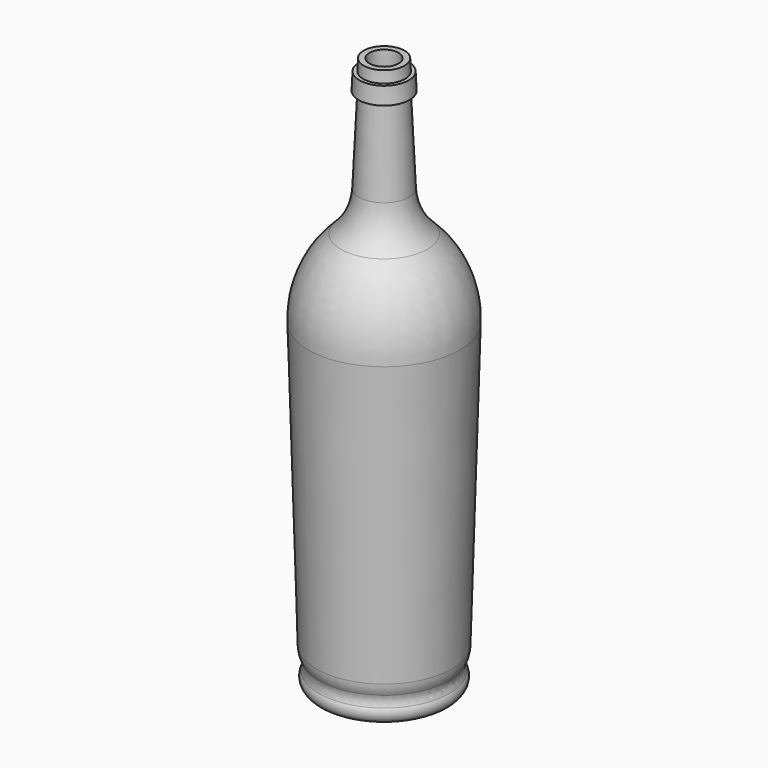
from build123d import *

# Parameters (mm, degrees)
F2_R = 1
F3_T = -0.5


with BuildPart() as f1:
    # F0 (on Front) → F1 (revolve)
    with BuildSketch(Plane.XZ):
        with BuildLine():
            Line((1.744893219, 47.2681485116), (0, 47.2681485116))
            Line((0, 47.2681485116), (0, 0))
            Line((0, 0), (5.1215616986, 0))
            ThreePointArc((5.1215616986, 0), (5.6702853456, 0.8186125558), (5.1215616986, 1.6372251117))
            ThreePointArc((5.1215616986, 1.6372251117), (5.5899847523, 2.3465653626), (5.7700355537, 3.1773273367))
            Line((5.7700355537, 3.1773273367), (6.4565917837, 27.4051882573))
            ThreePointArc((6.4565917837, 27.4051882573), (5.7866417171, 31.0405728949), (3.6890737014, 34.0844294905))
            ThreePointArc((3.6890737014, 34.0844294905), (2.5772947918, 35.6353223548), (2.127496893, 37.4897772264))
            Line((2.127496893, 37.4897772264), (1.7901111066, 44.8263114386))
            Line((1.7901111066, 44.8263114386), (2.1750065152, 44.8263114386))
            Line((2.1750065152, 44.8263114386), (2.1079314457, 46.2848747853))
            Line((2.1079314457, 46.2848747853), (1.7901111066, 46.2848747853))
            Line((1.7901111066, 46.2848747853), (1.744893219, 47.2681485116))
        make_face()
    revolve(axis=Axis((0, 0, 23.6340742558), (0, 0, -1)))

    # F2
    f2_edges = [f1.edges().sort_by_distance(p)[0] for p in [
        (-5.121562, 0, 1.637225),
    ]]
    fillet(f2_edges, radius=F2_R)

    # F3
    f3_openings = [f1.faces().sort_by_distance(p)[0] for p in [
        (0, 0, 47.268149),
    ]]
    offset(amount=F3_T, openings=f3_openings, kind=Kind.INTERSECTION)


solid = f1.part
